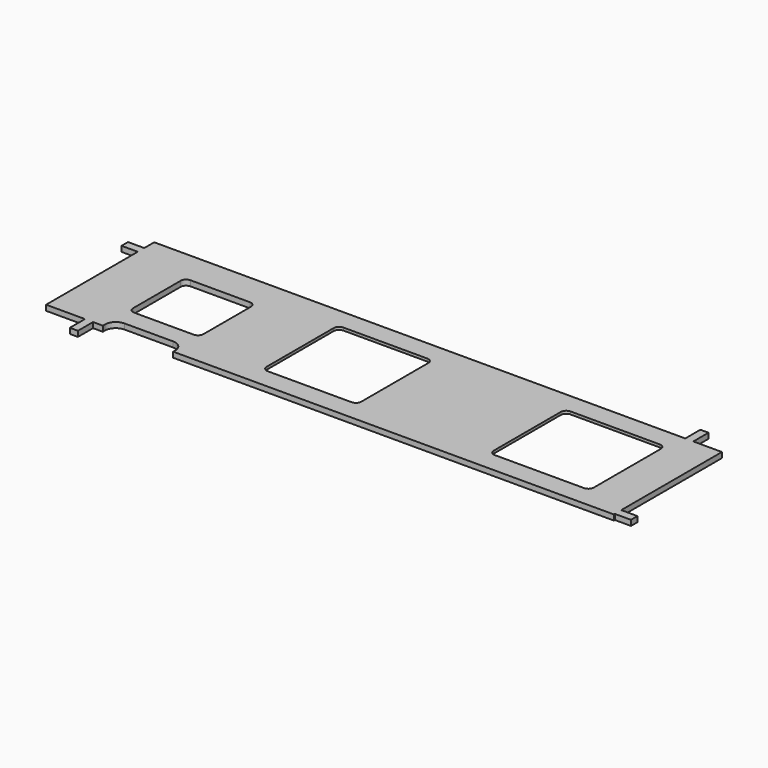
from build123d import *

# Parameters (mm, degrees)
F1_DEPTH  = 2
F2_W      = 26
F2_H      = 26
F3_DEPTH  = 15.4
F4_W      = 35
F4_H      = 35
F4_W_2    = 37
F5_DEPTH  = 25
F6_W      = 26
F6_H      = 5
F7_DEPTH  = 25
F8_R      = 4
F9_R      = 2
F10_W     = 46
F10_H     = 46
F10_W_2   = 48
F11_DEPTH = 1
F12_R     = 1
F13_R     = 1
F0_W      = 6
F0_H      = 3
F0_W_2    = 3
F0_H_2    = 7
F14_DEPTH = 2


# Not quite as in the source:
# - a feature names something its author has since deleted; it is built from what else it names


with BuildPart() as f1:
    # F0 (on Top) → F1 (new body)
    with BuildSketch(Plane.XY):
        Polygon((173.5389735401, 18.1442317292), (-22.8906879723, 18.1442317292), (-22.8906879723, 13.5384923518), (-22.8906879723, 10.5384923518), (-22.8906879723, -31.8557682708), (-8.5117332786, -31.8557682708), (-5.5117332786, -31.8557682708), (187.1093120277, -31.8557682708), (187.1093120277, -31.4002893865), (187.1093120277, -28.4002893865), (187.1093120277, 18.1442317292), (176.5389735401, 18.1442317292), align=None)
    extrude(amount=F1_DEPTH)

    # F2 (on face) → F3 (cut)
    with BuildSketch(Plane(origin=(0, 0, 0), x_dir=(1, 0, 0), z_dir=(0, 0, -1))):
        with Locations((11.1093120277, 6.8557682708)):
            Rectangle(F2_W, F2_H)
    extrude(amount=-F3_DEPTH, mode=Mode.SUBTRACT)

    # F4 (on face) → F5 (cut)
    with BuildSketch(Plane(origin=(0, 0, 0), x_dir=(1, 0, 0), z_dir=(0, 0, -1))):
        with Locations((68.6093120277, 6.8557682708)):
            Rectangle(F4_W, F4_H)
        with Locations((153.6093120277, 6.8557682708)):
            Rectangle(F4_W_2, F4_H)
    extrude(amount=-F5_DEPTH, mode=Mode.SUBTRACT)

    # F6 (on face) → F7 (cut)
    with BuildSketch(Plane.XY.offset(2)):
        with Locations((11.1093120277, -29.3557682708)):
            Rectangle(F6_W, F6_H)
    extrude(amount=-F7_DEPTH, mode=Mode.SUBTRACT)

    # F8
    f8_edges = [f1.edges().sort_by_distance(p)[0] for p in [
        (-1.890688, -26.855768, 1),
        (24.109312, -26.855768, 1),
    ]]
    fillet(f8_edges, radius=F8_R)

    # F9
    f9_edges = [f1.edges().sort_by_distance(p)[0] for p in [
        (51.109312, 10.644232, 1),
        (86.109312, 10.644232, 1),
        (51.109312, -24.355768, 1),
        (135.109312, -24.355768, 1),
        (86.109312, -24.355768, 1),
        (172.109312, -24.355768, 1),
        (135.109312, 10.644232, 1),
        (172.109312, 10.644232, 1),
        (24.109312, 6.144232, 1),
        (-1.890688, 6.144232, 1),
        (24.109312, -19.855768, 1),
        (-1.890688, -19.855768, 1),
    ]]
    fillet(f9_edges, radius=F9_R)

    # F10 (on face) → F11 (cut)
    with BuildSketch(Plane.XY):
        with Locations((68.6093120277, -6.8557682708)):
            Rectangle(F10_W, F10_H)
        with Locations((153.6093120277, -6.8557682708)):
            Rectangle(F10_W_2, F10_H)
    extrude(amount=F11_DEPTH, mode=Mode.SUBTRACT)

    # F12
    f12_edges = [f1.edges().sort_by_distance(p)[0] for p in [
        (45.609312, -29.855768, 0.5),
        (91.609312, -29.855768, 0.5),
        (91.609312, 16.144232, 0.5),
        (45.609312, 16.144232, 0.5),
    ]]
    fillet(f12_edges, radius=F12_R)

    # F13
    f13_edges = [f1.edges().sort_by_distance(p)[0] for p in [
        (129.609312, -29.855768, 0.5),
        (177.609312, -29.855768, 0.5),
        (177.609312, 16.144232, 0.5),
        (129.609312, 16.144232, 0.5),
    ]]
    fillet(f13_edges, radius=F13_R)

    # F0 (on Top) → F14 (join)
    with BuildSketch(Plane.XY):
        with Locations((190.1093120277, -29.9002893865)):
            Rectangle(F0_W, F0_H)
        with Locations((175.0389735401, 21.6442317292)):
            Rectangle(F0_W_2, F0_H_2)
        with Locations((-7.0117332786, -35.3557682708)):
            Rectangle(F0_W_2, F0_H_2)
        with Locations((-25.8906879723, 12.0384923518)):
            Rectangle(F0_W, F0_H)
    extrude(amount=F14_DEPTH)


solid = f1.part
